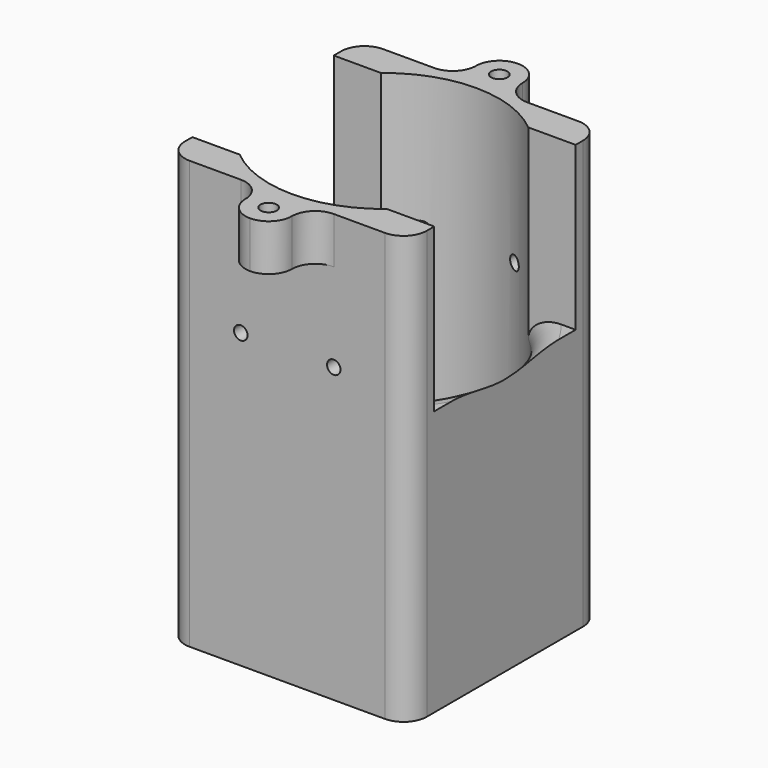
from build123d import *

# Parameters (mm, degrees)
F0_W         = 52
F0_H         = 52
F0_R         = 24.7301056407
F1_DEPTH     = 92
F2_W         = 38
F2_H         = 35
F3_DEPTH     = 52.001
F4_R         = 5
F5_T4_ANGLE  = 79.1651275765
F5_T9_ANGLE  = 158.3519759407
F5_T15_ANGLE = 79.1651275765
F6_R         = 1.45
F7_DEPTH     = 10
F8_R         = 1.45
F9_DEPTH     = 52.001
F10_W        = 25
F10_H        = 26
F11_DEPTH    = 92.0010001
F12_W        = 10
F12_H        = 10
F12_R        = 1.75
F13_DEPTH    = 10
F14_R        = 4.99999
F15_R        = 3
F16_DEPTH    = 4


# Not quite as in the source:
# - a fillet or chamfer that OpenCascade refuses, or shapes differently, is made with other operations: its cross-section is extruded or revolved along the edge and cut away or added
# - a fillet or chamfer is up to 0.001 mm smaller than in the source, because OpenCascade refuses the exact size


with BuildPart() as f1:
    # F0 (on Top) → F1 (new body)
    with BuildSketch(Plane.XY):
        Rectangle(F0_W, F0_H)
        Circle(F0_R, mode=Mode.SUBTRACT)
    extrude(amount=F1_DEPTH)

    # F2 (on face) → F3 (cut, through all)
    with BuildSketch(Plane(origin=(-26, 0, 0), x_dir=(0, -1, 0), z_dir=(-1, 0, 0))):
        with Locations((0, 74.5)):
            Rectangle(F2_W, F2_H)
    extrude(amount=-F3_DEPTH, mode=Mode.SUBTRACT)

    # F4
    f4_edges = [f1.edges().sort_by_distance(p)[0] for p in [
        (-26, 26, 46),
        (-26, -26, 46),
        (26, 26, 46),
        (26, -26, 46),
    ]]
    fillet(f4_edges, radius=F4_R)

    # F5: fillet of radius 5 on 3 edges, made by hand


with BuildPart() as f5_tool2:
    # F5_s3 → F5_t4 (revolve)
    with BuildSketch(Plane.XZ):
        with BuildLine():
            ThreePointArc((24.7301056407, 52), (26.1945717348, 55.5355339059), (29.7301056407, 57))
            Line((29.7301056407, 57), (24.7301056407, 57))
            Line((24.7301056407, 57), (24.7301056407, 52))
        make_face()
    revolve(axis=Axis((0, 0, 57), (0, 0, -1)), revolution_arc=F5_T4_ANGLE)

    split(bisect_by=Plane.XZ.offset(19), keep=Keep.BOTTOM)


with BuildPart() as f1_1:
    add(f1.part)

    # F5_t1: cut F5_tool2
    add(f5_tool2.part, mode=Mode.SUBTRACT)


with BuildPart() as f5_tool7:
    # F5_s8 → F5_t9 (revolve)
    with BuildSketch(Plane(origin=(0, 0, 0), x_dir=(0, 0, 1), z_dir=(0.982208635, -0.1877929639, 0))):
        with BuildLine():
            ThreePointArc((52, 24.7301056407), (55.5355339059, 26.1945717348), (57, 29.7301056407))
            Line((57, 29.7301056407), (57, 24.7301056407))
            Line((57, 24.7301056407), (52, 24.7301056407))
        make_face()
    revolve(axis=Axis((0, 0, 57), (0, 0, -1)), revolution_arc=F5_T9_ANGLE)

    split(bisect_by=Plane.XZ.offset(-19), keep=Keep.TOP)

    split(bisect_by=Plane.XZ.offset(19), keep=Keep.BOTTOM)


with BuildPart() as f1_2:
    add(f1_1.part)

    # F5_t6: cut F5_tool7
    add(f5_tool7.part, mode=Mode.SUBTRACT)


with BuildPart() as f5_tool13:
    # F5_s14 → F5_t15 (revolve)
    with BuildSketch(Plane(origin=(0, 0, 0), x_dir=(0, 0, 1), z_dir=(-0.9821730213, 0.1879791378, 0))):
        with BuildLine():
            ThreePointArc((52, 24.7301056407), (55.5355339059, 26.1945717348), (57, 29.7301056407))
            Line((57, 29.7301056407), (57, 24.7301056407))
            Line((57, 24.7301056407), (52, 24.7301056407))
        make_face()
    revolve(axis=Axis((0, 0, 57), (0, 0, -1)), revolution_arc=F5_T15_ANGLE)

    split(bisect_by=Plane.XZ.offset(-19), keep=Keep.TOP)


with BuildPart() as f1_3:
    add(f1_2.part)

    # F5_t12: cut F5_tool13
    add(f5_tool13.part, mode=Mode.SUBTRACT)

    # F6 (on face) → F7 (cut)
    with BuildSketch(Plane.XY):
        with Locations((-20, -20)):
            Circle(F6_R)
        with Locations((20, -20)):
            Circle(F6_R)
        with Locations((20, 20)):
            Circle(F6_R)
        with Locations((-20, 20)):
            Circle(F6_R)
    extrude(amount=F7_DEPTH, mode=Mode.SUBTRACT)

    # F8 (on face) → F9 (cut, through all)
    with BuildSketch(Plane(origin=(0, 26, 0), x_dir=(-1, 0, 0), z_dir=(0, 1, 0))):
        with Locations((-10, 63)):
            Circle(F8_R)
        with Locations((10, 63)):
            Circle(F8_R)
    extrude(amount=-F9_DEPTH, mode=Mode.SUBTRACT)

    # F10 (on face) → F11 (cut, through all)
    with BuildSketch(Plane.XY):
        with Locations((-28.625, 0)):
            Rectangle(F10_W, F10_H)
    extrude(amount=F11_DEPTH, mode=Mode.SUBTRACT)

    # F12 (on face) → F13 (join)
    with BuildSketch(Plane.XY.offset(92)):
        with Locations((0, -31)):
            Rectangle(F12_W, F12_H)
        with Locations((0, -31)):
            Circle(F12_R, mode=Mode.SUBTRACT)
        with Locations((0, 31)):
            Rectangle(F12_W, F12_H)
        with Locations((0, 31)):
            Circle(F12_R, mode=Mode.SUBTRACT)
    extrude(amount=-F13_DEPTH)

    # F14 (radius 5 in the source; OpenCascade refuses exactly that, so slightly less here)
    f14_edges = [f1_3.edges().sort_by_distance(p)[0] for p in [
        (-5, -26, 87),
        (5, -26, 87),
        (-5, 26, 87),
        (5, 26, 87),
        (5, 36, 87),
        (-5, 36, 87),
        (-5, -36, 87),
        (5, -36, 87),
    ]]
    fillet(f14_edges, radius=F14_R)

    # F15 (on face) → F16 (cut)
    with BuildSketch(Plane(origin=(0, 0, 82), x_dir=(1, 0, 0), z_dir=(0, 0, -1))):
        with Locations((0, 31.0749467462)):
            Circle(F15_R)
        with Locations((0, -31)):
            Circle(F15_R)
    extrude(amount=-F16_DEPTH, mode=Mode.SUBTRACT)


solid = f1_3.part
